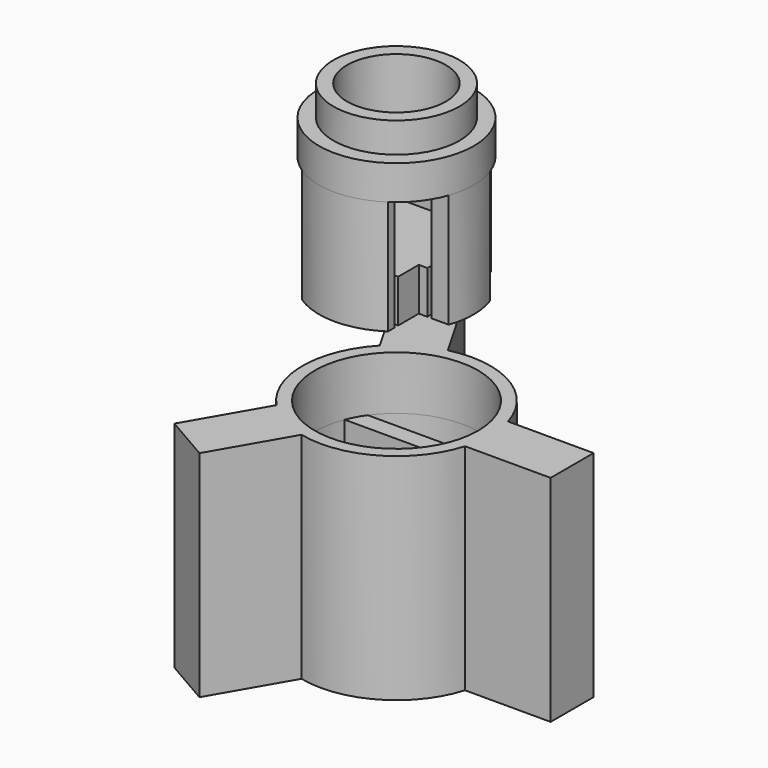
from build123d import *

# Parameters (mm, degrees)
F0_R      = 4.572
F0_R_2    = 2.921
F1_DEPTH  = 3.81
F2_R      = 4.572
F2_R_2    = 3.7211
F3_DEPTH  = 1.778
F5_DEPTH  = 3.556
F6_DEPTH  = 3.175
F8_DEPTH  = 2.54
F11_DEPTH = 6.35
F13_DEPTH = 3.175
F14_R     = 4.824416
F15_DEPTH = 3.175


# Not quite as in the source:
# - after a boolean that leaves OpenCascade's solid faulty, fix() repairs it


with BuildPart() as f1:
    # F0 (on Top) → F1 (new body)
    with BuildSketch(Plane.XY):
        Circle(F0_R)
        Circle(F0_R_2, mode=Mode.SUBTRACT)
    extrude(amount=F1_DEPTH)

    # F2 (on face) → F3 (cut)
    with BuildSketch(Plane.XY.offset(3.81)):
        Circle(F2_R)
        Circle(F2_R_2, mode=Mode.SUBTRACT)
    extrude(amount=-F3_DEPTH, mode=Mode.SUBTRACT)

    # F4 (on face) → F5 (join)
    with BuildSketch(Plane(origin=(0, 0, 0), x_dir=(1, 0, 0), z_dir=(0, 0, -1))):
        with BuildLine():
            Line((-3.302, 1.524), (-4.310523, 1.524))
            ThreePointArc((-4.310523, 1.524), (-4.572, 0), (-4.310523, -1.524))
            Line((-4.310523, -1.524), (-3.302, -1.524))
            Line((-3.302, -1.524), (-3.302, 1.524))
        make_face()
        with BuildLine():
            Line((-2.54, 3.302), (2.54, 3.302))
            Line((2.54, 3.302), (2.54, 3.801524))
            ThreePointArc((2.54, 3.801524), (0, 4.572), (-2.54, 3.801524))
            Line((-2.54, 3.801524), (-2.54, 3.302))
        make_face()
        with BuildLine():
            Line((4.310523, 1.524), (3.302, 1.524))
            Line((3.302, 1.524), (3.302, -1.524))
            Line((3.302, -1.524), (4.310523, -1.524))
            ThreePointArc((4.310523, -1.524), (4.572, 0), (4.310523, 1.524))
        make_face()
        with BuildLine():
            Line((2.54, -3.801524), (2.54, -3.302))
            Line((2.54, -3.302), (-2.54, -3.302))
            Line((-2.54, -3.302), (-2.54, -3.801524))
            ThreePointArc((-2.54, -3.801524), (0, -4.572), (2.54, -3.801524))
        make_face()
    extrude(amount=F5_DEPTH)

    add(f1.part.fix(), mode=Mode.REPLACE)

    # F6 (add): faces of the model
    f6_faces = [f1.faces().sort_by_distance(p)[0] for p in [
        (0, 3.838335, -3.556),
        (0, -3.838335, -3.556),
        (-3.896476, 0, -3.556),
        (3.896476, 0, -3.556),
    ]]
    extrude(f6_faces, amount=F6_DEPTH)


with BuildPart() as f8:
    # F7 (on face) → F8 (new body)
    with BuildSketch(Plane(origin=(0, 0, -6.731), x_dir=(1, 0, 0), z_dir=(0, 0, -1))):
        Polygon((-2.54, 1.524), (-3.048, 1.524), (-3.048, -1.524), (-2.54, -1.524), (-2.54, -3.048), (2.54, -3.048), (2.54, -1.524), (3.048, -1.524), (3.048, 1.524), (2.54, 1.524), (2.54, 3.048), (-2.54, 3.048), align=None)
    extrude(amount=-F8_DEPTH)


with BuildPart() as f11:
    # F10 (on offset) → F11 (new body)
    with BuildSketch(Plane.XY.offset(-25.4)):
        with BuildLine():
            Line((-6.56594, 8.197542), (-4.037134, 3.817521))
            ThreePointArc((-4.037134, 3.817521), (-5.55625, 0), (-4.037134, -3.817521))
            Line((-4.037134, -3.817521), (-6.56594, -8.197542))
            Line((-6.56594, -8.197542), (-3.81631, -9.785042))
            Line((-3.81631, -9.785042), (-1.287503, -5.405021))
            ThreePointArc((-1.287503, -5.405021), (2.778125, -4.811854), (5.324637, -1.5875))
            Line((5.324637, -1.5875), (10.38225, -1.5875))
            Line((10.38225, -1.5875), (10.38225, 1.5875))
            Line((10.38225, 1.5875), (5.324637, 1.5875))
            ThreePointArc((5.324637, 1.5875), (2.778125, 4.811854), (-1.287503, 5.405021))
            Line((-1.287503, 5.405021), (-3.81631, 9.785042))
            Line((-3.81631, 9.785042), (-6.56594, 8.197542))
        make_face()
        with BuildLine():
            ThreePointArc((2.794, -3.933008), (0, -4.824416), (-2.794, -3.933008))
            Line((-2.794, -3.933008), (-2.794, -2.794))
            Line((-2.794, -2.794), (2.794, -2.794))
            Line((2.794, -2.794), (2.794, -3.933008))
        make_face(mode=Mode.SUBTRACT)
        with BuildLine():
            Line((-4.485003, 1.777565), (-2.792902, 1.777565))
            Line((-2.792902, 1.777565), (-2.792902, -1.777565))
            Line((-2.792902, -1.777565), (-4.485003, -1.777565))
            ThreePointArc((-4.485003, -1.777565), (-4.824416, 0), (-4.485003, 1.777565))
        make_face(mode=Mode.SUBTRACT)
        with BuildLine():
            Line((2.794, 2.794), (-2.794, 2.794))
            Line((-2.794, 2.794), (-2.794, 3.933008))
            ThreePointArc((-2.794, 3.933008), (0, 4.824416), (2.794, 3.933008))
            Line((2.794, 3.933008), (2.794, 2.794))
        make_face(mode=Mode.SUBTRACT)
        with BuildLine():
            Line((4.485003, -1.777565), (2.792902, -1.777565))
            Line((2.792902, -1.777565), (2.792902, 1.777565))
            Line((2.792902, 1.777565), (4.485003, 1.777565))
            ThreePointArc((4.485003, 1.777565), (4.824416, 0), (4.485003, -1.777565))
        make_face(mode=Mode.SUBTRACT)
    extrude(amount=F11_DEPTH)

    # F12 (on face) → F13 (join)
    with BuildSketch(Plane.XY.offset(-19.05)):
        with BuildLine():
            Line((10.38225, -1.5875), (10.38225, 1.5875))
            Line((10.38225, 1.5875), (5.324637, 1.5875))
            ThreePointArc((5.324637, 1.5875), (2.778125, 4.811854), (-1.287503, 5.405021))
            Line((-1.287503, 5.405021), (-3.81631, 9.785042))
            Line((-3.81631, 9.785042), (-6.56594, 8.197542))
            Line((-6.56594, 8.197542), (-4.037134, 3.817521))
            ThreePointArc((-4.037134, 3.817521), (-5.55625, 0), (-4.037134, -3.817521))
            Line((-4.037134, -3.817521), (-6.56594, -8.197542))
            Line((-6.56594, -8.197542), (-3.81631, -9.785042))
            Line((-3.81631, -9.785042), (-1.287503, -5.405021))
            ThreePointArc((-1.287503, -5.405021), (2.778125, -4.811854), (5.324637, -1.5875))
            Line((5.324637, -1.5875), (10.38225, -1.5875))
        make_face()
        with BuildLine():
            ThreePointArc((3.933008, -2.794), (0, -4.824416), (-3.933008, -2.794))
            Line((-3.933008, -2.794), (3.933008, -2.794))
        make_face(mode=Mode.SUBTRACT)
        with BuildLine():
            Line((4.485003, -1.777565), (-4.485003, -1.777565))
            ThreePointArc((-4.485003, -1.777565), (-4.824416, 0), (-4.485003, 1.777565))
            Line((-4.485003, 1.777565), (4.485003, 1.777565))
            ThreePointArc((4.485003, 1.777565), (4.824416, 0), (4.485003, -1.777565))
        make_face(mode=Mode.SUBTRACT)
        with BuildLine():
            Line((3.933008, 2.794), (-3.933008, 2.794))
            ThreePointArc((-3.933008, 2.794), (0, 4.824416), (3.933008, 2.794))
        make_face(mode=Mode.SUBTRACT)
    extrude(amount=F13_DEPTH)

    # F14 (on face) → F15 (join)
    with BuildSketch(Plane.XY.offset(-15.875)):
        with BuildLine():
            Line((10.38225, -1.5875), (10.38225, 1.5875))
            Line((10.38225, 1.5875), (5.324637, 1.5875))
            ThreePointArc((5.324637, 1.5875), (2.778125, 4.811854), (-1.287503, 5.405021))
            Line((-1.287503, 5.405021), (-3.81631, 9.785042))
            Line((-3.81631, 9.785042), (-6.56594, 8.197542))
            Line((-6.56594, 8.197542), (-4.037134, 3.817521))
            ThreePointArc((-4.037134, 3.817521), (-5.55625, 0), (-4.037134, -3.817521))
            Line((-4.037134, -3.817521), (-6.56594, -8.197542))
            Line((-6.56594, -8.197542), (-3.81631, -9.785042))
            Line((-3.81631, -9.785042), (-1.287503, -5.405021))
            ThreePointArc((-1.287503, -5.405021), (2.778125, -4.811854), (5.324637, -1.5875))
            Line((5.324637, -1.5875), (10.38225, -1.5875))
        make_face()
        Circle(F14_R, mode=Mode.SUBTRACT)
    extrude(amount=F15_DEPTH)


solid = Compound([f1.part, f8.part, f11.part])
